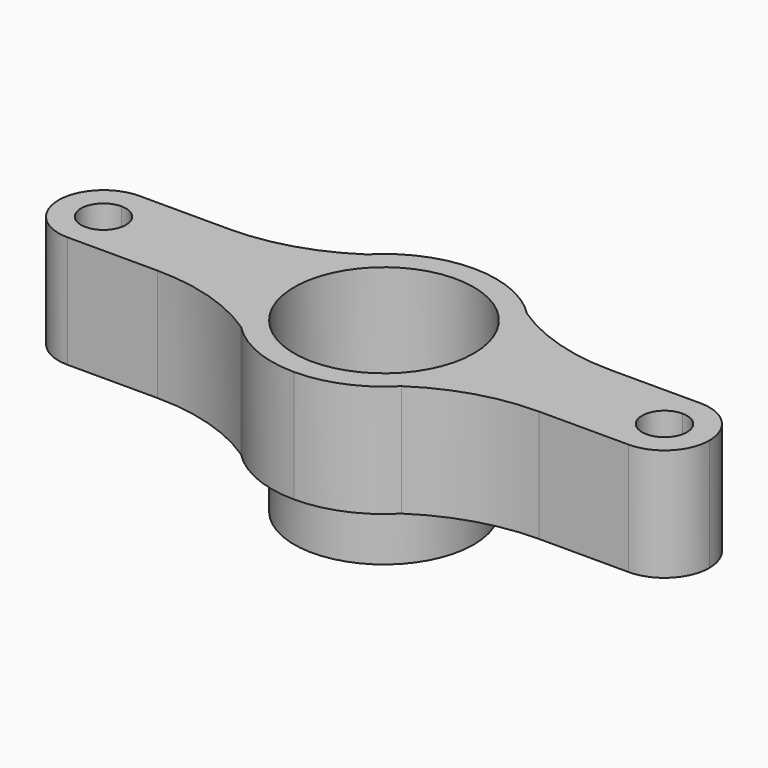
from build123d import *

# Parameters (mm, degrees)
F1_DEPTH = 10
F2_R     = 8
F3_DEPTH = 15
F4_R     = 8
F5_DEPTH = 10
F6_R     = 3
F7_DEPTH = 25


with BuildPart() as f1:
    # F0 (on Top) → F1 (new body)
    with BuildSketch(Plane.XY):
        with BuildLine():
            Line((-25, 2), (-25, 4))
            ThreePointArc((-25, 4), (-29, 0), (-25, -4))
            Line((-25, -4), (-25, -2))
            ThreePointArc((-25, -2), (-27, 0), (-25, 2))
        make_face()
        with BuildLine():
            ThreePointArc((-21, 0), (-22.1715728753, 2.8284271247), (-25, 4))
            Line((-25, 4), (-25, 2))
            ThreePointArc((-25, 2), (-23.5857864376, 1.4142135624), (-23, 0))
            ThreePointArc((-23, 0), (-23.5857864376, -1.4142135624), (-25, -2))
            Line((-25, -2), (-25, -4))
            ThreePointArc((-25, -4), (-22.1715728753, -2.8284271247), (-21, 0))
        make_face()
        with BuildLine():
            ThreePointArc((-7.1414284285, -7), (-10, 0), (-7.1414284285, 7))
            ThreePointArc((-7.1414284285, 7), (-11.8475386118, 4.7666024499), (-17, 4))
            Line((-17, 4), (-25, 4))
            ThreePointArc((-25, 4), (-22.1715728753, 2.8284271247), (-21, 0))
            ThreePointArc((-21, 0), (-22.1715728753, -2.8284271247), (-25, -4))
            Line((-25, -4), (-17, -4))
            ThreePointArc((-17, -4), (-11.8475386118, -4.7666024499), (-7.1414284285, -7))
        make_face()
        with BuildLine():
            Line((-2.6925824036, 7), (-7.1414284285, 7))
            ThreePointArc((-7.1414284285, 7), (-10, 0), (-7.1414284285, -7))
            Line((-7.1414284285, -7), (-2.6925824036, -7))
            ThreePointArc((-2.6925824036, -7), (-7.5, 0), (-2.6925824036, 7))
        make_face()
        with BuildLine():
            ThreePointArc((7.1414284285, -7), (9.2578151927, -3.7805896177), (10, 0))
            ThreePointArc((10, 0), (9.2578151927, 3.7805896177), (7.1414284285, 7))
            Line((7.1414284285, 7), (2.6925824036, 7))
            ThreePointArc((2.6925824036, 7), (6.1824092402, 4.2459175671), (7.5, 0))
            ThreePointArc((7.5, 0), (6.1824092402, -4.2459175671), (2.6925824036, -7))
            Line((2.6925824036, -7), (7.1414284285, -7))
        make_face()
        with BuildLine():
            ThreePointArc((7.1414284285, 7), (9.2578151927, 3.7805896177), (10, 0))
            ThreePointArc((10, 0), (9.2578151927, -3.7805896177), (7.1414284285, -7))
            ThreePointArc((7.1414284285, -7), (11.8475386118, -4.7666024499), (17, -4))
            Line((17, -4), (25, -4))
            ThreePointArc((25, -4), (21, 0), (25, 4))
            Line((25, 4), (17, 4))
            ThreePointArc((17, 4), (11.8475386118, 4.7666024499), (7.1414284285, 7))
        make_face()
        with BuildLine():
            ThreePointArc((-2.6925824036, -7), (-1.3693063938, -7.3739406019), (0, -7.5))
            Line((0, -7.5), (0, -7))
            Line((0, -7), (-2.6925824036, -7))
        make_face()
        with BuildLine():
            ThreePointArc((0, -7.5), (1.3693063938, -7.3739406019), (2.6925824036, -7))
            Line((2.6925824036, -7), (0, -7))
            Line((0, -7), (0, -7.5))
        make_face()
        with BuildLine():
            ThreePointArc((-7.1414284285, -7), (-3.8729833462, -9.2195444573), (0, -10))
            Line((0, -10), (0, -7.5))
            ThreePointArc((0, -7.5), (-1.3693063938, -7.3739406019), (-2.6925824036, -7))
            Line((-2.6925824036, -7), (-7.1414284285, -7))
        make_face()
        with BuildLine():
            ThreePointArc((0, -10), (3.8729833462, -9.2195444573), (7.1414284285, -7))
            Line((7.1414284285, -7), (2.6925824036, -7))
            ThreePointArc((2.6925824036, -7), (1.3693063938, -7.3739406019), (0, -7.5))
            Line((0, -7.5), (0, -10))
        make_face()
        with BuildLine():
            Line((0, 3), (0, 7))
            Line((0, 7), (-2.6925824036, 7))
            ThreePointArc((-2.6925824036, 7), (-7.5, 0), (-2.6925824036, -7))
            Line((-2.6925824036, -7), (0, -7))
            Line((0, -7), (0, -3))
            ThreePointArc((0, -3), (-3, 0), (0, 3))
        make_face()
        with BuildLine():
            ThreePointArc((7.5, 0), (6.1824092402, 4.2459175671), (2.6925824036, 7))
            Line((2.6925824036, 7), (0, 7))
            Line((0, 7), (0, 3))
            ThreePointArc((0, 3), (2.1213203436, 2.1213203436), (3, 0))
            ThreePointArc((3, 0), (2.1213203436, -2.1213203436), (0, -3))
            Line((0, -3), (0, -7))
            Line((0, -7), (2.6925824036, -7))
            ThreePointArc((2.6925824036, -7), (6.1824092402, -4.2459175671), (7.5, 0))
        make_face()
        with BuildLine():
            Line((25, 2), (25, 4))
            ThreePointArc((25, 4), (21, 0), (25, -4))
            Line((25, -4), (25, -2))
            ThreePointArc((25, -2), (23, 0), (25, 2))
        make_face()
        with BuildLine():
            ThreePointArc((29, 0), (27.8284271247, 2.8284271247), (25, 4))
            Line((25, 4), (25, 2))
            ThreePointArc((25, 2), (26.4142135624, 1.4142135624), (27, 0))
            ThreePointArc((27, 0), (26.4142135624, -1.4142135624), (25, -2))
            Line((25, -2), (25, -4))
            ThreePointArc((25, -4), (27.8284271247, -2.8284271247), (29, 0))
        make_face()
        with BuildLine():
            Line((0, 7), (0, 7.5))
            ThreePointArc((0, 7.5), (-1.3693063938, 7.3739406019), (-2.6925824036, 7))
            Line((-2.6925824036, 7), (0, 7))
        make_face()
        with BuildLine():
            Line((0, 7), (2.6925824036, 7))
            ThreePointArc((2.6925824036, 7), (1.3693063938, 7.3739406019), (0, 7.5))
            Line((0, 7.5), (0, 7))
        make_face()
        with BuildLine():
            Line((0, 7.5), (0, 10))
            ThreePointArc((0, 10), (-3.8729833462, 9.2195444573), (-7.1414284285, 7))
            Line((-7.1414284285, 7), (-2.6925824036, 7))
            ThreePointArc((-2.6925824036, 7), (-1.3693063938, 7.3739406019), (0, 7.5))
        make_face()
        with BuildLine():
            Line((2.6925824036, 7), (7.1414284285, 7))
            ThreePointArc((7.1414284285, 7), (3.8729833462, 9.2195444573), (0, 10))
            Line((0, 10), (0, 7.5))
            ThreePointArc((0, 7.5), (1.3693063938, 7.3739406019), (2.6925824036, 7))
        make_face()
    extrude(amount=F1_DEPTH)


with BuildPart() as f3:
    # F2 (on face) → F3 (new body)
    with BuildSketch(Plane.XY.offset(10)):
        Circle(F2_R)
    extrude(amount=-F3_DEPTH)


with BuildPart() as f5_tool:
    # F4 (on face) → F5 (new body)
    with BuildSketch(Plane.XY.offset(10)):
        Circle(F4_R)
    extrude(amount=-F5_DEPTH)


with BuildPart() as f1_1:
    add(f1.part)

    # F5: cut by f5_tool
    add(f5_tool.part, mode=Mode.SUBTRACT)


with BuildPart() as f3_1:
    add(f3.part)

    # F5: cut by f5_tool
    add(f5_tool.part, mode=Mode.SUBTRACT)

    # F6 (on Top) → F7 (cut)
    with BuildSketch(Plane.XY):
        Circle(F6_R)
    extrude(amount=-F7_DEPTH, mode=Mode.SUBTRACT)


solid = Compound([f1_1.part, f3_1.part])
